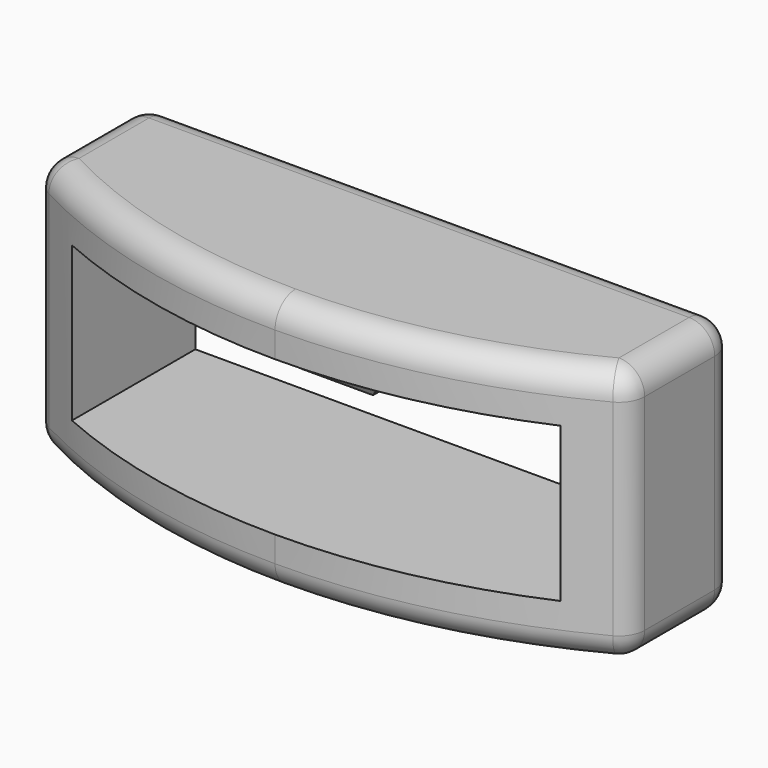
from build123d import *

# Parameters (mm, degrees)
F0_W     = 23
F0_H     = 10
F1_DEPTH = 4
F3_DEPTH = 10.001
F4_W     = 19
F4_H     = 6
F5_DEPTH = 8.001
F6_W     = 6
F6_H     = 4
F8_W     = 2.8015887365
F8_H     = 1.9735014066
F11_R    = 1


# Not quite as in the source:
# - a feature of the source that left no trace in its solid (it failed there, or was rolled back) is left out


with BuildPart() as f1:
    # F0 (on Front) → F1 (new body, symmetric)
    with BuildSketch(Plane.XZ):
        Rectangle(F0_W, F0_H)
    extrude(amount=F1_DEPTH, both=True)

    # F2 (on face) → F3 (cut, through all)
    with BuildSketch(Plane.XY.offset(5)):
        with BuildLine():
            ThreePointArc((-6.62e-08, -4), (-5.9424321941, -3.2376566126), (-11.5, -1))
            Line((-11.5, -1), (-11.5, -4))
            Line((-11.5, -4), (-6.62e-08, -4))
        make_face()
        with BuildLine():
            ThreePointArc((11.5, -1), (5.94243213, -3.2376566294), (-6.62e-08, -4))
            Line((-6.62e-08, -4), (11.5, -4))
            Line((11.5, -4), (11.5, -1))
        make_face()
    extrude(amount=-F3_DEPTH, mode=Mode.SUBTRACT)

    # F4 (on face) → F5 (cut, through all)
    with BuildSketch(Plane(origin=(0, 4, 0), x_dir=(-1, 0, 0), z_dir=(0, 1, 0))):
        Rectangle(F4_W, F4_H)
    extrude(amount=-F5_DEPTH, mode=Mode.SUBTRACT)

    # F6 (on face) → F9 section 0
    with BuildSketch(Plane(origin=(0, 0, 3), x_dir=(1, 0, 0), z_dir=(0, 0, -1))):
        Rectangle(F6_W, F6_H)
    # F8 (on offset) → F9 section 1
    with BuildSketch(Plane(origin=(0, 0, 1), x_dir=(1, 0, 0), z_dir=(0, 0, -1))):
        Rectangle(F8_W, F8_H)
    loft()

    # F11
    f11_edges = [f1.edges().sort_by_distance(p)[0] for p in [
        (11.5, 1.5, -5),
        (-11.5, 1.5, -5),
        (11.5, 1.5, 5),
        (-11.5, 1.5, 5),
        (11.5, -1, 0),
        (11.5, 4, 0),
        (0, 4, -5),
        (0, -4, -5),
        (0, -4, 5),
        (-11.5, -1, 0),
        (0, 4, 5),
        (-11.5, 4, 0),
    ]]
    fillet(f11_edges, radius=F11_R)


solid = f1.part
